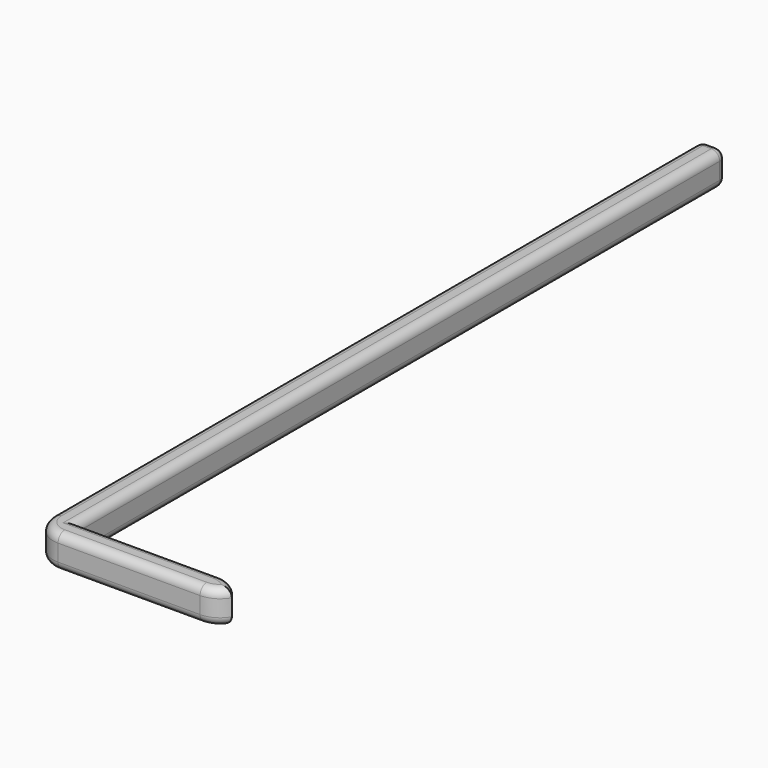
from build123d import *

# Parameters (mm, degrees)
F1_DEPTH    = 2
F2_T1_DEPTH = 9.5
F3_R        = 0.5


# Not quite as in the source:
# - a fillet or chamfer that OpenCascade refuses, or shapes differently, is made with other operations: its cross-section is extruded or revolved along the edge and cut away or added


with BuildPart() as f1:
    # F0 (on Top) → F1 (new body)
    with BuildSketch(Plane.XY):
        Polygon((1.5, 0), (0, 0), (0, -50), (11.5, -50), (11.5, -48.5), (1.5, -48.5), align=None)
    extrude(amount=F1_DEPTH)

    # F2: fillet of radius 1.5 on 3 edges, made by hand

    # F2_s2 → F2_t1 (cut)
    with BuildSketch(Plane.XY.offset(-3.75)):
        with BuildLine():
            ThreePointArc((10, -50), (11.0606601718, -49.5606601718), (11.5, -48.5))
            Line((11.5, -48.5), (11.5, -50))
            Line((11.5, -50), (10, -50))
        make_face()
        with BuildLine():
            ThreePointArc((0, -48.5), (0.4393398282, -49.5606601718), (1.5, -50))
            Line((1.5, -50), (0, -50))
            Line((0, -50), (0, -48.5))
        make_face()
        with BuildLine():
            ThreePointArc((11.5, -50), (11.0606601718, -48.9393398282), (10, -48.5))
            Line((10, -48.5), (11.5, -48.5))
            Line((11.5, -48.5), (11.5, -50))
        make_face()
    extrude(amount=F2_T1_DEPTH, mode=Mode.SUBTRACT)

    # F3
    f3_edges = [f1.edges().sort_by_distance(p)[0] for p in [
        (0, -24.25, 2),
        (0, -24.25, 0),
        (1.5, -24.25, 0),
        (1.5, -24.25, 2),
        (1.5, 0, 1),
        (0, 0, 1),
        (0.75, 0, 0),
        (0.75, 0, 2),
        (5.75, -48.5, 0),
        (10.75, -48.700962, 0),
        (10.75, -49.799038, 0),
        (5.75, -50, 0),
        (0.43934, -49.56066, 0),
        (5.75, -48.5, 2),
        (10.75, -48.700962, 2),
        (10.75, -49.799038, 2),
        (5.75, -50, 2),
        (0.43934, -49.56066, 2),
    ]]
    fillet(f3_edges, radius=F3_R)


solid = f1.part
